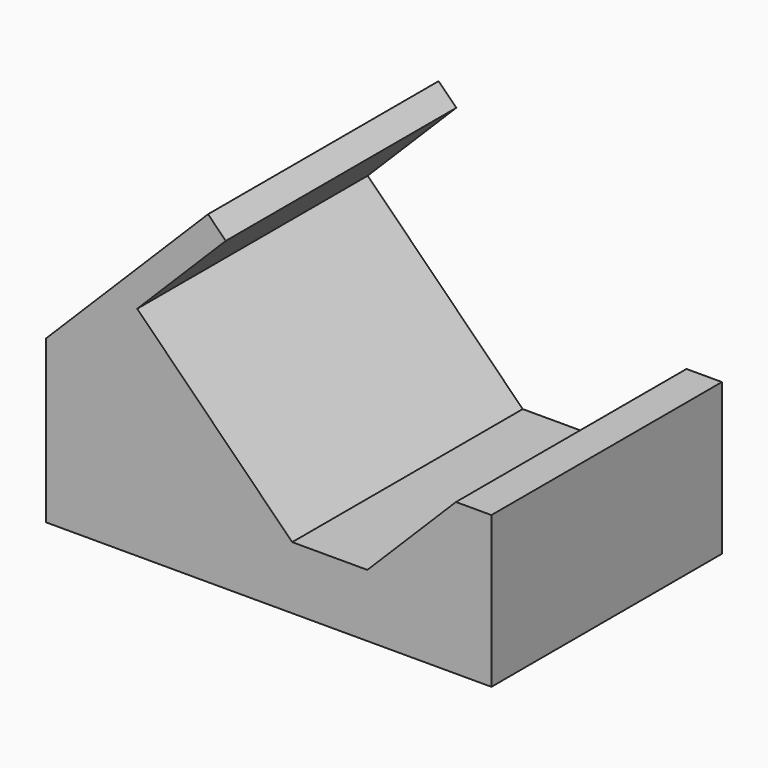
from build123d import *

# Parameters (mm, degrees)
F1_DEPTH = 46


# Not quite as in the source:
# - a feature names something its author has since deleted; it is built from what else it names


with BuildPart() as f1:
    # F0 (on Front) → F1 (new body)
    with BuildSketch(Plane.XZ):
        Polygon((54.1421356237, 14.1421356237), (40, 0), (28, 0), (3.2512626585, 24.7487373415), (17.3933982822, 38.8908729653), (14.5649711575, 41.71930009), (-11.2946788875, 15.859650045), (-11.2946788875, -10), (59.7989898732, -10), (59.7989898732, 14.1421356237), align=None)
    extrude(amount=F1_DEPTH)


solid = f1.part
